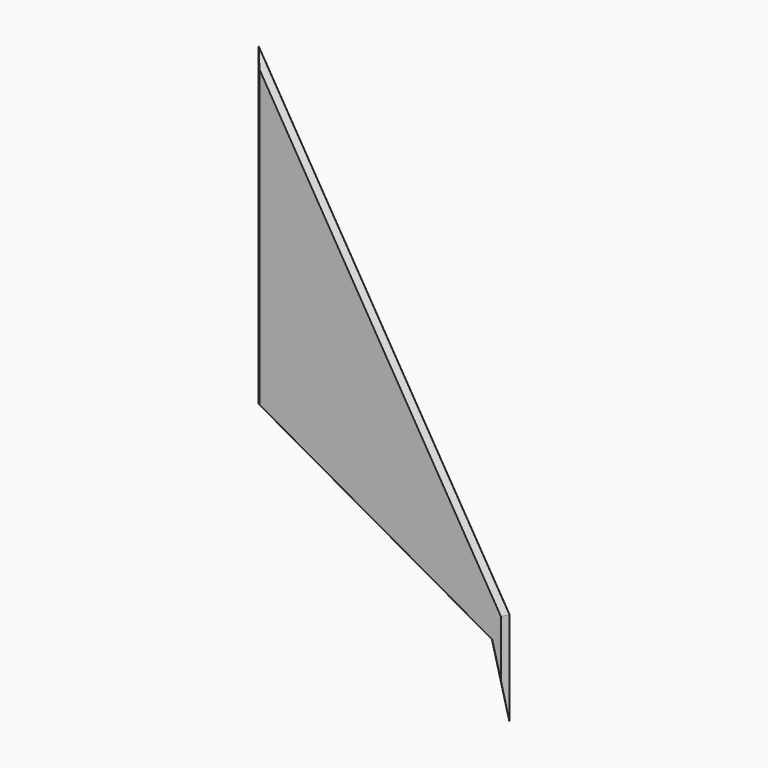
from build123d import *

# Parameters (mm, degrees)
F1_DEPTH = 3.81
F2_SIZE  = 1.90499


# Not quite as in the source:
# - a fillet or chamfer is up to 0.001 mm smaller than in the source, because OpenCascade refuses the exact size


with BuildPart() as f1:
    # F0 (on Front) → F1 (new body)
    with BuildSketch(Plane.XZ):
        Polygon((101.1442430278, -75.9420931081), (0, 92.935864608), (0, -34.064135392), (94.0731655183, -87.0116757444), (101.1442430278, -114.0420931081), align=None)
    extrude(amount=F1_DEPTH)

    # F2 (size 1.905 in the source; OpenCascade refuses exactly that, so slightly less here)
    f2_edges = [f1.edges().sort_by_distance(p)[0] for p in [
        (47.036583, -3.81, -60.537906),
        (97.608704, -3.81, -100.526884),
        (101.144243, -3.81, -94.992093),
        (50.572122, -3.81, 8.496886),
        (0, -3.81, 29.435865),
        (47.036583, 0, -60.537906),
        (97.608704, 0, -100.526884),
        (101.144243, 0, -94.992093),
        (50.572122, 0, 8.496886),
        (0, 0, 29.435865),
    ]]
    chamfer(f2_edges, length=F2_SIZE)


solid = f1.part
